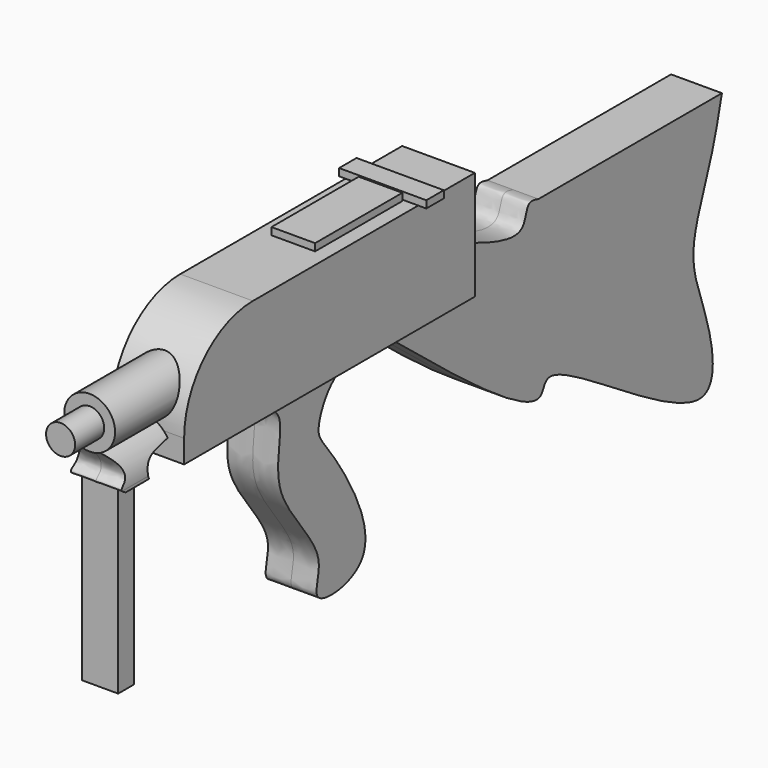
from build123d import *

# Parameters (mm, degrees)
F0_W         = 50
F0_H         = 15
F4_DEPTH     = 5
F6_DEPTH     = 3.5
F7_DEPTH     = 3.5
F8_R         = 3.5
F9_DEPTH     = 10
F11_DEPTH    = 3.5
F12_T4_DEPTH = 31.1925308579
F12_T9_DEPTH = 31.1925308579
F13_W        = 2.6911012828
F13_H        = 25.6362333894
F14_DEPTH    = 2.5
F16_W        = 10
F16_H        = 3
F16_W_2      = 0.8856946416
F16_W_3      = 1.1143053584
F17_DEPTH    = 1
F15_W        = 6
F15_H        = 15
F18_DEPTH    = 1
F19_R        = 2
F20_DEPTH    = 5
F23_T4_DEPTH = 69.1482322781
F23_S5_R     = 3.5
F23_T6_DEPTH = 37


# Not quite as in the source:
# - a fillet or chamfer that OpenCascade refuses, or shapes differently, is made with other operations: its cross-section is extruded or revolved along the edge and cut away or added
# - the program builds the solid bodies; features that only make, move or delete a surface that nothing else refers to are left out


with BuildPart() as f4:
    # F0 (on Right) → F4 (new body, symmetric)
    with BuildSketch(Plane.YZ):
        Rectangle(F0_W, F0_H)
    extrude(amount=F4_DEPTH, both=True)

    # F1 (on Right) → F6 (join, symmetric)
    with BuildSketch(Plane.YZ):
        with BuildLine():
            add(Edge.make_bspline(
                [(5.0288359635, -7.4090333655), (3.8747425174, -8.0396121547), (1.5058055584, -9.333962629), (-0.6659366061, -14.3473039029), (1.7900139344, -16.7150092177), (13.3298427925, -34.3338449276), (-2.5168468775, -35.6944299553), (2.3604454281, -28.8366802251), (-9.3580369544, -19.2293074855), (-5.1281425989, -9.3300178953), (-8.7157958407, -7.8506437555), (-10.2017633617, -7.2379028425)],
                knots=[0, 0, 0, 0, 0.085060873, 0.1745992463, 0.2560750759, 0.4269788129, 0.5453812336, 0.634660935, 0.7886330355, 0.9124540687, 1, 1, 1, 1], degree=3))
            Line((5.0288359635, -7.4090333655), (-10.2017633617, -7.2379028425))
        make_face()
    extrude(amount=F6_DEPTH, both=True)

    # F3 (on Right) → F7 (join, symmetric)
    with BuildSketch(Plane.YZ):
        with BuildLine():
            Line((24.7045550495, -7.2819935158), (11.484448798, -7.2819930501))
            add(Edge.make_bspline(
                [(11.484448798, -7.2819930501), (23.6117533605, -17.0911157265), (39.0057683758, -29.5425043256), (38.4769679365, -19.4731144784), (69.7511129966, -44.8764958695), (67.2652908622, -27.1730877398), (62.9400583518, -19.2390483674), (67.5136212356, -9.3788074704), (68.7710991059, -3.9630220268), (69.3724676967, -1.3730096398)],
                knots=[0, 0, 0, 0, 0.2299750996, 0.2919230831, 0.5106876233, 0.6280997743, 0.7557988233, 0.8832147102, 1, 1, 1, 1], degree=3))
            Line((69.3724676967, -1.3730096398), (37.8245003521, -1.3730096398))
            add(Edge.make_bspline(
                [(37.8245003521, -1.3730096398), (37.1580512672, -1.187243061), (35.6543126329, -0.7680896887), (35.6692021274, -5.8469046645), (29.0798478957, -3.1582564204), (24.7045550495, -1.3730096398)],
                knots=[0, 0, 0, 0, 0.2110125183, 0.4761169057, 1, 1, 1, 1], degree=3))
            Line((24.7045550495, -1.3730096398), (24.7045550495, -7.2819935158))
        make_face()
    extrude(amount=F7_DEPTH, both=True)

    # F8 (on face) → F9 (join, symmetric)
    with BuildSketch(Plane.XZ.offset(25)):
        Circle(F8_R)
    extrude(amount=F9_DEPTH, both=True)

    # F10 (on Right) → F11 (join, symmetric)
    with BuildSketch(Plane.YZ):
        with BuildLine():
            add(Edge.make_bspline(
                [(-25.0070467591, -5.0111194141), (-25.9612180154, -5.1341997717), (-27.703561445, -5.3531032437), (-29.3504881217, -6.1384351315), (-29.4547779314, -7.411750037), (-29.1655181944, -8.0482149497)],
                knots=[0, 0, 0, 0, 0.3925157934, 0.6905923264, 1, 1, 1, 1], degree=3))
            Line((-25.0070467591, -5.0111194141), (-25.0721182674, -3.3436943777))
            Line((-25.0721182674, -3.3436943777), (-34.7138419747, -3.3436943777))
            add(Edge.make_bspline(
                [(-33.1655181944, -8.0482149497), (-33.5320342546, -7.8562966256), (-34.2967631965, -7.4558626123), (-32.8675088407, -6.6927583961), (-33.0520601488, -5.2273844056), (-33.9244570896, -4.1725097863), (-34.45901522, -3.6112499704), (-34.7138419747, -3.3436943777)],
                knots=[0, 0, 0, 0, 0.1787892659, 0.3730404776, 0.5852209013, 0.8022725582, 1, 1, 1, 1], degree=3))
            Line((-33.1655181944, -8.0482149497), (-29.1655181944, -8.0482149497))
        make_face()
    extrude(amount=F11_DEPTH, both=True)

    # F12: fillet of radius 5 on 2 edges, made by hand


with BuildPart() as f12_tool2:
    # F12_s3 → F12_t4 (new body)
    with BuildSketch(Plane.XZ.offset(14.2967146921)):
        with BuildLine():
            ThreePointArc((1.0342668459, -3.3436943777), (2.8400077321, -5.1710483475), (3.5, -7.6538558078))
            Line((3.5, -7.6538558078), (3.5, -3.3436943777))
            Line((3.5, -3.3436943777), (1.0342668459, -3.3436943777))
        make_face()
    extrude(amount=F12_T4_DEPTH)

    split(bisect_by=Plane.XZ.offset(25), keep=Keep.TOP)


with BuildPart() as f4_1:
    add(f4.part)

    # F12_t1: cut F12_tool2
    add(f12_tool2.part, mode=Mode.SUBTRACT)


with BuildPart() as f12_tool7:
    # F12_s8 → F12_t9 (new body)
    with BuildSketch(Plane.XZ.offset(14.2967146921)):
        with BuildLine():
            ThreePointArc((-1.0342668459, -3.3436943777), (-2.8400077321, -5.1710483475), (-3.5, -7.6538558078))
            Line((-3.5, -7.6538558078), (-3.5, -3.3436943777))
            Line((-3.5, -3.3436943777), (-1.0342668459, -3.3436943777))
        make_face()
    extrude(amount=F12_T9_DEPTH)

    split(bisect_by=Plane.XZ.offset(25), keep=Keep.TOP)


with BuildPart() as f4_2:
    add(f4_1.part)

    # F12_t6: cut F12_tool7
    add(f12_tool7.part, mode=Mode.SUBTRACT)

    # F13 (on Right) → F14 (join, symmetric)
    with BuildSketch(Plane.YZ):
        with Locations((-31.8762697279, -19.9134759605)):
            Rectangle(F13_W, F13_H)
    extrude(amount=F14_DEPTH, both=True)

    # F16 (on face) → F17 (join)
    with BuildSketch(Plane.XY.offset(7.5)):
        with Locations((0, 16.7606703341)):
            Rectangle(F16_W, F16_H)
        with Locations((-5.4428473208, 16.7606703341)):
            Rectangle(F16_W_2, F16_H)
        with Locations((5.5571526792, 16.7606703341)):
            Rectangle(F16_W_3, F16_H)
    extrude(amount=F17_DEPTH)

    # F15 (on face) → F18 (join)
    with BuildSketch(Plane.XY.offset(7.5)):
        with Locations((0.0187216531, 7.5)):
            Rectangle(F15_W, F15_H)
    extrude(amount=F18_DEPTH)

    # F19 (on face) → F20 (join)
    with BuildSketch(Plane.XZ.offset(35)):
        Circle(F19_R)
    extrude(amount=F20_DEPTH)

    # F23: fillet of radius 11.8296464556 on 1 edges, made by hand


with BuildPart() as f23_tool2:
    # F23_s3 → F23_t4 (new body)
    with BuildSketch(Plane.YZ.offset(34.5741161391)):
        with BuildLine():
            ThreePointArc((-25, -4.3296464556), (-21.5351767722, 4.0351767722), (-13.1703535444, 7.5))
            Line((-13.1703535444, 7.5), (-25, 7.5))
            Line((-25, 7.5), (-25, -4.3296464556))
        make_face()
    extrude(amount=-F23_T4_DEPTH)

    # F23_s5 → F23_t6 (cut, symmetric)
    with BuildSketch(Plane.XZ.offset(19.1)):
        Circle(F23_S5_R)
    extrude(amount=F23_T6_DEPTH, both=True, mode=Mode.SUBTRACT)


with BuildPart() as f4_3:
    add(f4_2.part)

    # F23_t1: cut F23_tool2
    add(f23_tool2.part, mode=Mode.SUBTRACT)


solid = f4_3.part
